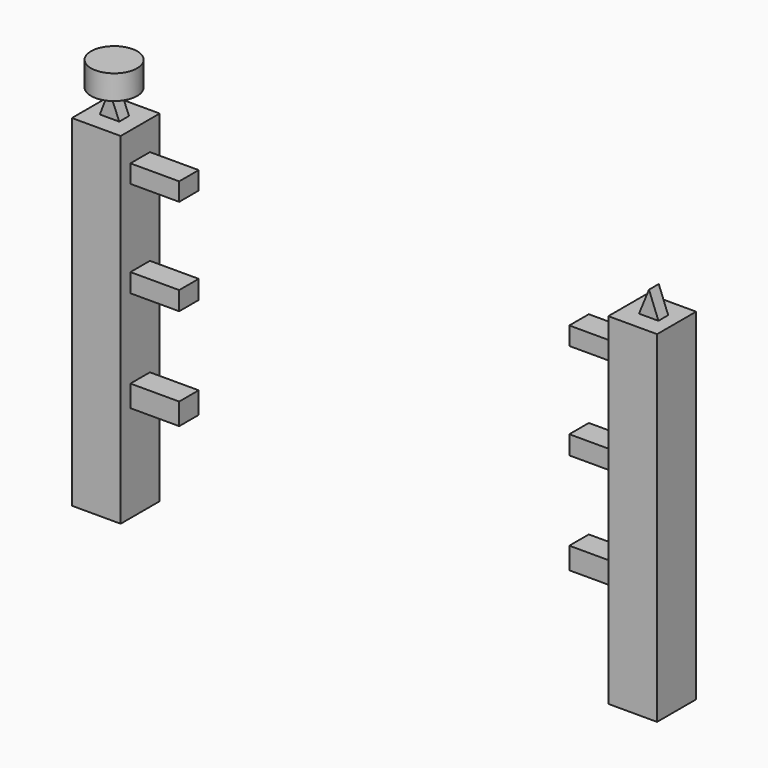
from build123d import *

# Parameters (mm, degrees)
F1_DEPTH = 6.35
F0_W     = 12.7
F0_H     = 4.7037045424
F0_H_2   = 4.8604938446
F0_H_3   = 5.6444450735
F2_DEPTH = 3.175
F0_W_2   = 6.0121872838
F0_H_4   = 6.35
F4_DEPTH = 1.5875


with BuildPart() as f1:
    # F0 (on Front) → F1 (new body, symmetric)
    with BuildSketch(Plane.XZ):
        Polygon((-76.2, -56.4129777904), (-63.5, -56.4129777904), (-63.5, -31.2012367346), (-63.5, -25.5567916611), (-63.5, -4.8604938446), (-63.5, 0), (-63.5, 20.2259261356), (-63.5, 24.929630678), (-63.5, 32.4870222096), (-67.6794573665, 32.4870222096), (-72.7410018444, 32.4870222096), (-76.2, 32.4870222096), align=None)
    extrude(amount=F1_DEPTH, both=True)

    # F0 (on Front) → F2 (join, symmetric)
    with BuildSketch(Plane.XZ):
        with Locations((-57.15, 22.5777784068)):
            Rectangle(F0_W, F0_H)
        with Locations((-57.15, -2.4302469223)):
            Rectangle(F0_W, F0_H_2)
        with Locations((-57.15, -28.3790141978)):
            Rectangle(F0_W, F0_H_3)
    extrude(amount=F2_DEPTH, both=True)

    # F0 (on Front) → F4 (join, symmetric)
    with BuildSketch(Plane.XZ):
        Polygon((-70.2845623006, 38.8370222096), (-72.7410018444, 32.4870222096), (-67.6794573665, 32.4870222096), align=None)
    extrude(amount=F4_DEPTH, both=True)


with BuildPart() as f3:
    # F0 (on Front) → F3 (revolve)
    with BuildSketch(Plane.XZ):
        with Locations((-67.2784686587, 42.0120222096)):
            Rectangle(F0_W_2, F0_H_4)
    revolve(axis=Axis((-70.2845623006, 0, 42.0120222096), (0, 0, -1)))


with BuildPart() as f5_1:
    # F5: instance of F1
    add(f1.part.mirror(Plane.YZ))


solid = Compound([f1.part, f3.part, f5_1.part])
